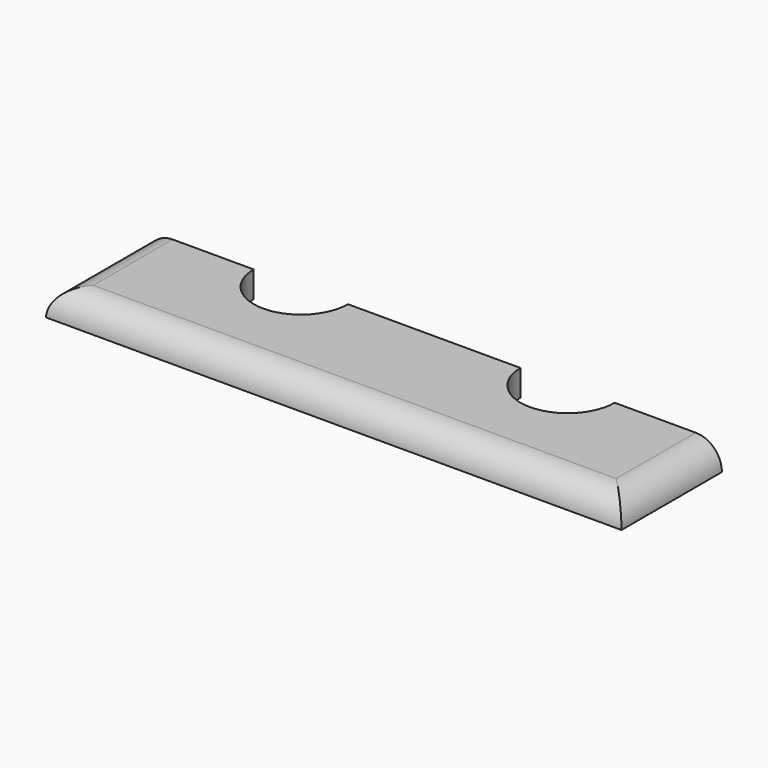
from build123d import *

# Parameters (mm, degrees)
F1_DEPTH = 5
F2_R     = 4.99999


# Not quite as in the source:
# - a fillet or chamfer is up to 0.001 mm smaller than in the source, because OpenCascade refuses the exact size


with BuildPart() as f1:
    # F0 (on Top) → F1 (new body)
    with BuildSketch(Plane.XY):
        with BuildLine():
            Line((16.5, 0), (0, 0))
            Line((0, 0), (-16.5, 0))
            ThreePointArc((-16.5, 0), (-25.5, -9), (-34.5, 0))
            Line((-34.5, 0), (-55, 0))
            Line((-55, 0), (-55, -24))
            Line((-55, -24), (0, -24))
            Line((0, -24), (55, -24))
            Line((55, -24), (55, 0))
            Line((55, 0), (34.5, 0))
            ThreePointArc((34.5, 0), (25.5, -9), (16.5, 0))
        make_face()
    extrude(amount=F1_DEPTH)

    # F2 (radius 5 in the source; OpenCascade refuses exactly that, so slightly less here)
    f2_edges = [f1.edges().sort_by_distance(p)[0] for p in [
        (0, -24, 5),
        (-55, -12, 5),
        (55, -12, 5),
    ]]
    fillet(f2_edges, radius=F2_R)


solid = f1.part
